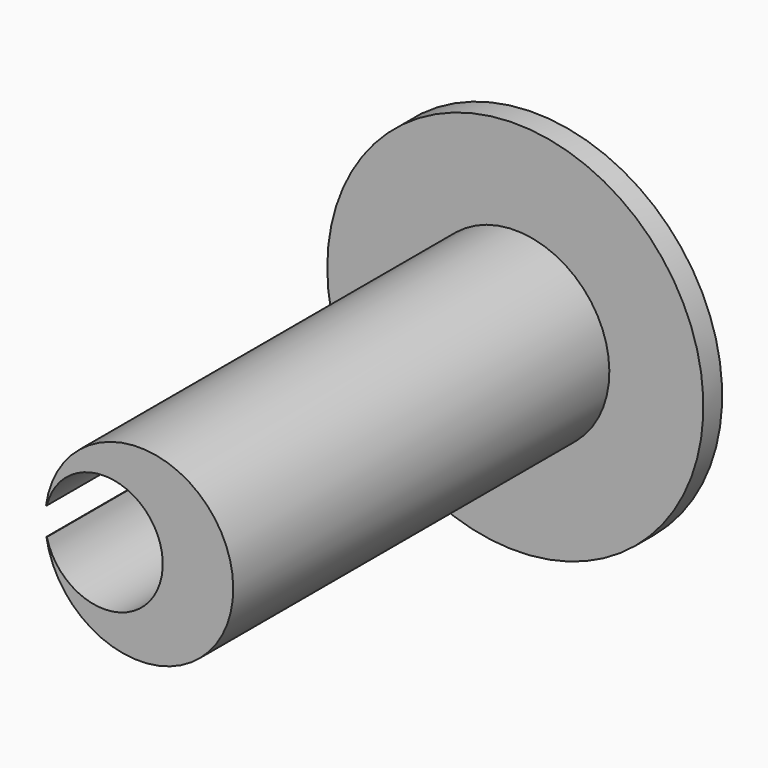
from build123d import *
from build123d import SkipClean  # not in build123d's __all__

# Parameters (mm, degrees)
F1_DEPTH = 21
F2_R     = 8
F3_DEPTH = 1


with BuildPart() as f1:
    # F0 (on Front) → F1 (new body)
    with BuildSketch(Plane.XZ):
        with BuildLine():
            Line((-3.928567067, -0.6374265649), (-3.9488843202, -0.6374265649))
            ThreePointArc((-3.9488843202, -0.6374265649), (3.9997163197, 0.0476378244), (-3.9629458697, 0.5431942877))
            Line((-3.9629458697, 0.5431942877), (-3.928567067, 0.5431942877))
            ThreePointArc((-3.928567067, 0.5431942877), (1.0007401595, -0.0471161386), (-3.928567067, -0.6374265649))
        make_face()
    extrude(amount=F1_DEPTH)

    # F2 (on face) → F3 (join)
    with BuildSketch(Plane(origin=(0, 0, 0), x_dir=(-1, 0, 0), z_dir=(0, 1, 0))):
        Circle(F2_R)
        with BuildLine():
            ThreePointArc((3.928567067, 0.5431942877), (3.9815237333, 0.250147998), (3.9992598405, -0.0471161386))
            ThreePointArc((3.9992598405, -0.0471161386), (3.9815237333, -0.3443802752), (3.928567067, -0.6374265649))
            Line((3.928567067, -0.6374265649), (3.9488843202, -0.6374265649))
            ThreePointArc((3.9488843202, -0.6374265649), (-3.9997163197, 0.0476378244), (3.9629458697, 0.5431942877))
            Line((3.9629458697, 0.5431942877), (3.928567067, 0.5431942877))
        make_face(mode=Mode.SUBTRACT)
    with SkipClean():  # cleaning this boolean's faces spoils the solid; the shape is the same uncleaned
        extrude(amount=-F3_DEPTH)


solid = f1.part
